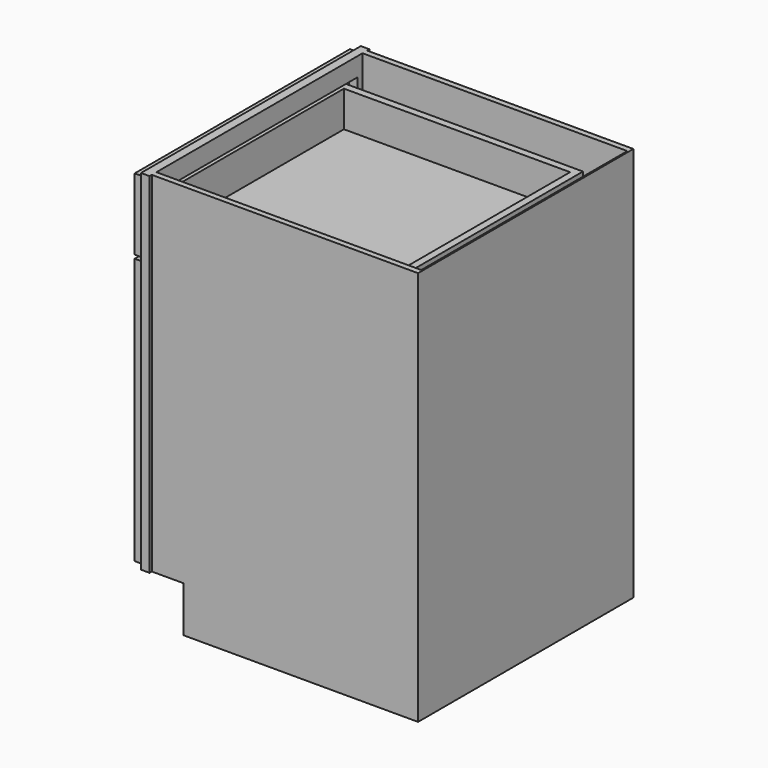
from build123d import *

# Parameters (mm, degrees)
F0_W          = 609.6
F0_H          = 876.3
F1_DEPTH      = 609.6
F2_W          = 88.9
F2_H          = 101.6
F3_DEPTH      = 609.601
F4_W          = 544.6426229508
F4_H          = 692.15
F5_DEPTH      = 19.05
F6_W          = 590.55
F6_H          = 6.35
F7_DEPTH      = 876.301
F8_W          = 587.375
F8_H          = 571.5
F9_DEPTH      = 733.425
F10_W         = 544.6426229508
F10_H         = 41.275
F11_DEPTH     = 19.05
F12_W         = 298.45
F12_H         = 590.5627
F12_W_2       = 184.15
F12_H_2       = 476.2627
F13_DEPTH     = 19.05
F14_W         = 6.35
F14_H         = 184.15
F15_DEPTH     = 476.2627
F16_SIZE      = 3.175
F17_W         = 596.9
F17_H         = 158.75
F17_W_2       = 482.6
F17_H_2       = 82.55
F18_DEPTH     = 19.05
F19_W         = 6.35
F19_H         = 482.6
F20_DEPTH     = 82.55
F21_SIZE      = 3.175
F22_W         = 504.825
F22_H         = 571.5
F23_DEPTH     = 101.6
F24_W         = 508
F24_H         = 95.25
F25_DEPTH     = 533.4
F26_T         = 15.875
F26_T3_DEPTH  = 37.249261314
F26_T5_DEPTH  = 37.249261314
F26_T7_DEPTH  = 37.249261314
F26_T9_DEPTH  = 37.249261314
F26_T11_DEPTH = 36.5125
F26_T13_DEPTH = 514.35
F26_T15_DEPTH = 114.3
F26_T17_DEPTH = 127
F26_T19_DEPTH = 539.75
F26_T21_DEPTH = 111.125
F26_T23_DEPTH = 36.5125


# Not quite as in the source:
# - a shell that OpenCascade refuses in one call is made with other operations: the cavity is built on its own and cut out


with BuildPart() as f1:
    # F0 (on Front) → F1 (new body)
    with BuildSketch(Plane.XZ):
        Rectangle(F0_W, F0_H)
    extrude(amount=-F1_DEPTH)

    # F2 (on face) → F3 (cut, through all)
    with BuildSketch(Plane.XZ):
        with Locations((-260.35, -387.35)):
            Rectangle(F2_W, F2_H)
    extrude(amount=-F3_DEPTH, mode=Mode.SUBTRACT)

    # F4 (on face) → F5 (cut)
    with BuildSketch(Plane(origin=(-304.8, 0, 0), x_dir=(0, -1, 0), z_dir=(-1, 0, 0))):
        with Locations((-304.8, 50.8)):
            Rectangle(F4_W, F4_H)
    extrude(amount=-F5_DEPTH, mode=Mode.SUBTRACT)

    # F6 (on face) → F7 (cut, through all)
    with BuildSketch(Plane.XY.offset(438.15)):
        with Locations((9.525, 606.425)):
            Rectangle(F6_W, F6_H)
        with Locations((9.525, 3.175)):
            Rectangle(F6_W, F6_H)
    extrude(amount=-F7_DEPTH, mode=Mode.SUBTRACT)

    # F8 (on face) → F9 (cut, through all)
    with BuildSketch(Plane.XY.offset(438.15)):
        with Locations((7.9375, 304.8)):
            Rectangle(F8_W, F8_H)
    extrude(amount=-F9_DEPTH, mode=Mode.SUBTRACT)

    # F10 (on face) → F11 (join, through all)
    with BuildSketch(Plane(origin=(-304.8, 0, 0), x_dir=(0, -1, 0), z_dir=(-1, 0, 0))):
        with Locations((-304.8, 265.1125)):
            Rectangle(F10_W, F10_H)
    extrude(amount=-F11_DEPTH)

    # F22 (on face) → F23 (cut)
    with BuildSketch(Plane(origin=(0, 0, -438.15), x_dir=(1, 0, 0), z_dir=(0, 0, -1))):
        with Locations((49.2125, -304.8)):
            Rectangle(F22_W, F22_H)
    extrude(amount=-F23_DEPTH, mode=Mode.SUBTRACT)


with BuildPart() as f13:
    # F12 (on face) → F13 (new body)
    with BuildSketch(Plane(origin=(-304.8, 0, 0), x_dir=(0, -1, 0), z_dir=(-1, 0, 0))):
        with Locations((-454.025, -33.33115)):
            Rectangle(F12_W, F12_H)
        with Locations((-454.025, -33.33115)):
            Rectangle(F12_W_2, F12_H_2, mode=Mode.SUBTRACT)
    extrude(amount=F13_DEPTH)

    # F14 (on face) → F15 (join, through all)
    with BuildSketch(Plane.XY.offset(-271.4625)):
        with Locations((-312.7375, 454.025)):
            Rectangle(F14_W, F14_H)
    extrude(amount=F15_DEPTH)

    # F16
    f16_edges = [f13.edges().sort_by_distance(p)[0] for p in [
        (-323.85, 546.1, -33.33115),
        (-323.85, 454.025, -271.4625),
        (-323.85, 361.95, -33.33115),
        (-323.85, 454.025, 204.8002),
    ]]
    chamfer(f16_edges, length=F16_SIZE)


with BuildPart() as f18:
    # F17 (on face) → F18 (new body)
    with BuildSketch(Plane(origin=(-304.8, 0, 0), x_dir=(0, -1, 0), z_dir=(-1, 0, 0))):
        with Locations((-304.8, 349.25)):
            Rectangle(F17_W, F17_H)
        with Locations((-304.8, 349.25)):
            Rectangle(F17_W_2, F17_H_2, mode=Mode.SUBTRACT)
    extrude(amount=F18_DEPTH)

    # F19 (on face) → F20 (join, through all)
    with BuildSketch(Plane.XY.offset(307.975)):
        with Locations((-312.7375, 304.8)):
            Rectangle(F19_W, F19_H)
    extrude(amount=F20_DEPTH)

    # F21
    f21_edges = [f18.edges().sort_by_distance(p)[0] for p in [
        (-323.85, 304.8, 307.975),
        (-323.85, 546.1, 349.25),
        (-323.85, 304.8, 390.525),
        (-323.85, 63.5, 349.25),
    ]]
    chamfer(f21_edges, length=F21_SIZE)

    # F24 (on face) → F25 (join)
    with BuildSketch(Plane.YZ.offset(-304.8)):
        with Locations((304.8, 339.725)):
            Rectangle(F24_W, F24_H)
    extrude(amount=F25_DEPTH)

    # F26: shell of thickness 15.875, made by hand


with BuildPart() as f26_core1:
    # F26_t2: copy of F18
    add(f18.part)

    # the walls: a layer under each face that stays
    f26_faces = [f26_core1.faces().sort_by_distance(p)[0] for p in [
        (-323.85, 503.7666666667, 296.3333333333),
        (-322.2625, 304.8, 306.3875),
        (-322.2625, 61.9125, 349.25),
        (-322.2625, 547.6875, 349.25),
        (-322.2625, 304.8, 392.1125),
        (-314.325, 304.8, 428.625),
        (-314.325, 603.25, 349.25),
        (-314.325, 304.8, 269.875),
        (-314.325, 6.35, 349.25),
        (-318.29375, 304.8, 307.975),
        (-318.29375, 63.5, 349.25),
        (-318.29375, 546.1, 349.25),
        (-318.29375, 304.8, 390.525),
        (-304.8, 503.7666666667, 402.1666666667),
        (-315.9125, 304.8, 349.25),
        (-38.1, 558.8, 339.725),
        (-38.1, 304.8, 292.1),
        (-38.1, 50.8, 339.725),
        (-307.18125, 63.5, 349.25),
        (-307.18125, 304.8, 390.525),
        (-307.18125, 546.1, 349.25),
        (-304.8, 304.8, 347.6625),
        (228.6, 304.8, 339.725),
        (-307.18125, 304.8, 307.975),
        (-309.5625, 304.8, 349.25),
    ]]
    thicken(f26_faces, amount=-F26_T, mode=Mode.SUBTRACT)

    # F26_s4 → F26_t3 (cut)
    with BuildSketch(Plane(origin=(4.5928978099, 4.5928978099, 4.5928978099), x_dir=(-0.7071067812, 0.7071067812, 0), z_dir=(0.5773502692, 0.5773502692, 0.5773502692))):
        Polygon((271.8908726623, 356.5892701441), (263.7152476623, 342.7036353262), (255.7777476623, 347.2863530879), (255.7777476623, 356.4517886113), align=None)
    extrude(amount=F26_T3_DEPTH, mode=Mode.SUBTRACT)

    # F26_s6 → F26_t5 (cut)
    with BuildSketch(Plane(origin=(-198.6071021901, 198.60710219, -198.6071021901), x_dir=(0.7071067812, 0.7071067812, 0), z_dir=(0.5773502692, -0.5773502692, 0.5773502692))):
        Polygon((159.161421149, 605.4574280109), (167.337046149, 591.571793193), (175.274546149, 596.1545109546), (175.274546149, 605.319946478), align=None)
    extrude(amount=F26_T5_DEPTH, mode=Mode.SUBTRACT)

    # F26_s8 → F26_t7 (cut)
    with BuildSketch(Plane(origin=(-228.2404355234, -228.2404355234, 228.2404355234), x_dir=(-0.7071067812, 0.7071067812, 0), z_dir=(0.5773502692, 0.5773502692, -0.5773502692))):
        Polygon((271.8908726623, 213.7335916339), (255.7777476623, 213.8710731668), (255.7777476623, 223.0365086901), (263.7152476623, 227.6192264518), align=None)
    extrude(amount=F26_T7_DEPTH, mode=Mode.SUBTRACT)

    # F26_s10 → F26_t9 (cut)
    with BuildSketch(Plane(origin=(-431.4404355234, 431.4404355234, 431.4404355234), x_dir=(0.7071067812, 0.7071067812, 0), z_dir=(0.5773502692, -0.5773502692, -0.5773502692))):
        Polygon((159.161421149, -35.1345662329), (175.274546149, -34.9970847), (175.274546149, -25.8316491766), (167.337046149, -21.2489314149), align=None)
    extrude(amount=F26_T9_DEPTH, mode=Mode.SUBTRACT)

    # F26_s12 → F26_t11 (cut)
    with BuildSketch(Plane.YZ.offset(-336.55)):
        Polygon((545.94125, 308.13375), (546.1, 292.1), (561.975, 292.1), (561.975, 307.975), align=None)
        Polygon((63.65875, 308.13375), (63.5, 292.1), (47.625, 292.1), (47.625, 307.975), align=None)
        Polygon((63.65875, 390.36625), (47.625, 390.525), (47.625, 406.4), (63.5, 406.4), align=None)
        Polygon((545.94125, 390.36625), (561.975, 390.525), (561.975, 406.4), (546.1, 406.4), align=None)
    extrude(amount=F26_T11_DEPTH, mode=Mode.SUBTRACT)

    # F26_s14 → F26_t13 (cut)
    with BuildSketch(Plane.XZ.offset(-561.975)):
        Polygon((-316.07125, 308.13375), (-315.9125, 292.1), (-300.0375, 292.1), (-300.0375, 307.975), align=None)
        Polygon((-316.07125, 390.36625), (-315.9125, 406.4), (-300.0375, 406.4), (-300.0375, 390.525), align=None)
        Polygon((-309.40375, 390.36625), (-309.5625, 406.4), (-325.4375, 406.4), (-325.4375, 390.525), align=None)
        Polygon((-304.95875, 308.13375), (-288.925, 307.975), (-288.925, 292.1), (-304.8, 292.1), align=None)
        Polygon((-309.40375, 308.13375), (-309.5625, 292.1), (-325.4375, 292.1), (-325.4375, 307.975), align=None)
    extrude(amount=F26_T13_DEPTH, mode=Mode.SUBTRACT)

    # F26_s16 → F26_t15 (cut)
    with BuildSketch(Plane.XY.offset(292.1)):
        Polygon((-316.07125, 63.65875), (-315.9125, 47.625), (-300.0375, 47.625), (-300.0375, 63.5), align=None)
        Polygon((-316.07125, 545.94125), (-315.9125, 561.975), (-300.0375, 561.975), (-300.0375, 546.1), align=None)
        Polygon((-309.40375, 63.65875), (-309.5625, 47.625), (-325.4375, 47.625), (-325.4375, 63.5), align=None)
        Polygon((-309.40375, 545.94125), (-309.5625, 561.975), (-325.4375, 561.975), (-325.4375, 546.1), align=None)
    extrude(amount=F26_T15_DEPTH, mode=Mode.SUBTRACT)

    # F26_s18 → F26_t17 (cut)
    with BuildSketch(Plane.XY.offset(276.225)):
        Polygon((-304.64125, 558.95875), (-320.675, 558.8), (-320.675, 542.925), (-304.8, 542.925), align=None)
        Polygon((-304.64125, 50.64125), (-320.675, 50.8), (-320.675, 66.675), (-304.8, 66.675), align=None)
    extrude(amount=F26_T17_DEPTH, mode=Mode.SUBTRACT)

    # F26_s20 → F26_t19 (cut)
    with BuildSketch(Plane.XZ.offset(-574.675)):
        Polygon((-304.64125, 291.94125), (-320.675, 292.1), (-320.675, 307.975), (-304.8, 307.975), align=None)
    extrude(amount=F26_T19_DEPTH, mode=Mode.SUBTRACT)

    # F26_s22 → F26_t21 (cut)
    with BuildSketch(Plane.XY.offset(292.1)):
        Polygon((-304.95875, 63.65875), (-304.8, 47.625), (-288.925, 47.625), (-288.925, 63.5), align=None)
        Polygon((-304.95875, 545.94125), (-304.8, 561.975), (-288.925, 561.975), (-288.925, 546.1), align=None)
    extrude(amount=F26_T21_DEPTH, mode=Mode.SUBTRACT)

    # F26_s24 → F26_t23 (cut)
    with BuildSketch(Plane.YZ.offset(-325.4375)):
        Polygon((63.65875, 308.13375), (47.625, 307.975), (47.625, 292.1), (63.5, 292.1), align=None)
        Polygon((63.65875, 390.36625), (47.625, 390.525), (47.625, 406.4), (63.5, 406.4), align=None)
        Polygon((545.94125, 390.36625), (546.1, 406.4), (561.975, 406.4), (561.975, 390.525), align=None)
        Polygon((545.94125, 308.13375), (561.975, 307.975), (561.975, 292.1), (546.1, 292.1), align=None)
    extrude(amount=F26_T23_DEPTH, mode=Mode.SUBTRACT)


with BuildPart() as f18_1:
    add(f18.part)

    # what is left inside the walls is the cavity
    f26_cavity = [f26_core1.part.solids().sort_by_distance(p)[0] for p in [
        (45.508333, 304.8, 308.13375),
    ]]
    add(f26_cavity, mode=Mode.SUBTRACT)


with BuildPart() as f27_1:
    # F27: instance of F13
    add(f13.part.mirror(Plane(origin=(-314.325, 304.8, -33.33115), x_dir=(1, 0, 0), z_dir=(0, -1, 0))))


solid = Compound([f1.part, f13.part, f18_1.part, f27_1.part])
